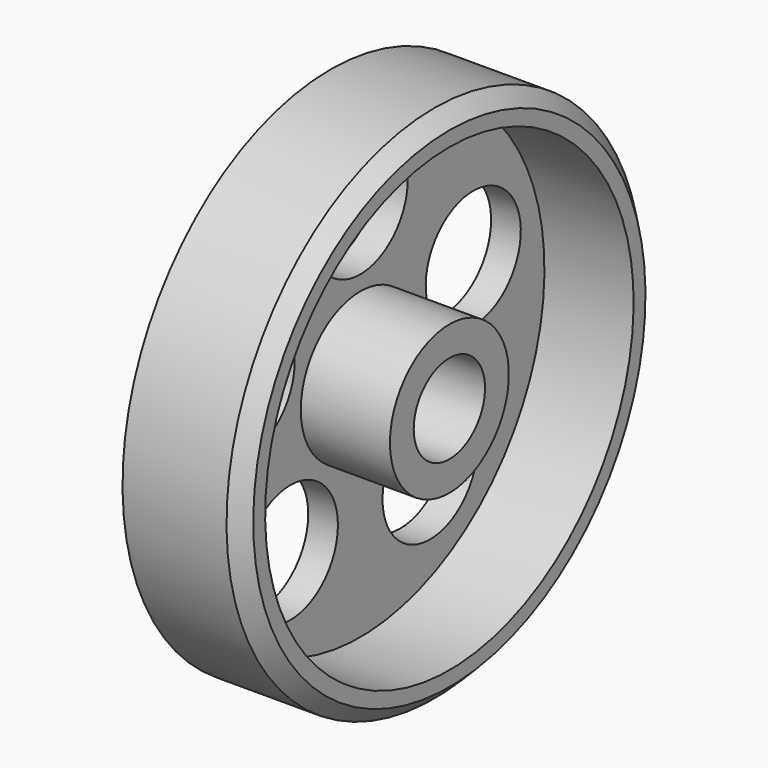
from build123d import *

# Parameters (mm, degrees)
F0_W            = 8
F0_H            = 17.5
F3_D            = 6
F4_T            = -2
F6_D            = 8
F6_COPIES_COUNT = 5
F7_SIZE         = 1


# Not quite as in the source:
# - a pattern or mirror of a feature is missing from the dataset's text; its kind, count and spacing are read off the source's solid


with BuildPart() as f1:
    # F0 (on Front) → F1 (revolve)
    with BuildSketch(Plane.XZ):
        with Locations((4, 8.75)):
            Rectangle(F0_W, F0_H)
    revolve(axis=Axis((4, 0, 0), (1, 0, 0)))

    # F3 (through all)
    with Locations(Plane(origin=(0, 0, 0), x_dir=(0, 1, 0), z_dir=(-1, 0, 0))):
        with Locations((0, 0)):
            Hole(F3_D / 2)

    # F4
    f4_openings = [f1.faces().sort_by_distance(p)[0] for p in [
        (8, 0, -17.005025),
    ]]
    offset(amount=F4_T, openings=f4_openings)

    # F6 (through all)
    with Locations(Plane(origin=(0, 0, 0), x_dir=(0, 1, 0), z_dir=(-1, 0, 0))):
        with Locations((0, -10)):
            f6 = Hole(F6_D / 2)

    # F6_copies: F6 ×5 about axis
    f6_copies_axis = Axis((0, 0, 0), (1, 0, 0))
    for i in range(1, F6_COPIES_COUNT):
        add(f6.rotate(f6_copies_axis, i * 360 / F6_COPIES_COUNT), mode=Mode.SUBTRACT)

    # F7
    f7_edges = [f1.edges().sort_by_distance(p)[0] for p in [
        (8, 0, -17.5),
    ]]
    chamfer(f7_edges, length=F7_SIZE)


solid = f1.part
